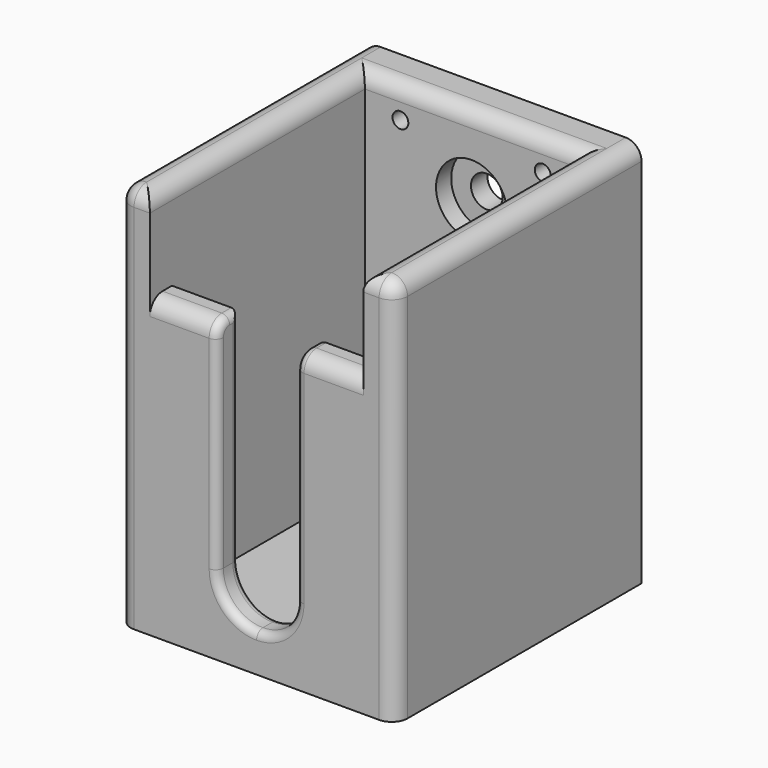
from build123d import *

# Parameters (mm, degrees)
F0_W           = 9
F0_H           = 7.5
F0_W_2         = 13.5
F0_H_2         = 34.5
F1_DEPTH       = 39
F2_DEPTH       = 34
F3_D           = 2
F3_DEPTH       = 40
F3_START       = 34
F3_TIP         = 0.600860619
F4_DEPTH       = 3.5
F5_R           = 1.99999
F7_D           = 4
F7_DEPTH       = 10
F7_CBORE_D     = 9
F7_CBORE_DEPTH = 2.4
F7_TIP         = 1.2017212381
F8_DEPTH       = 50
F9_R           = 1


# Not quite as in the source:
# - a fillet or chamfer is up to 0.001 mm smaller than in the source, because OpenCascade refuses the exact size


with BuildPart() as f1:
    # F0 (on Front) → F1 (new body)
    with BuildSketch(Plane.XZ):
        Polygon((13.5, 0), (0, 0), (-13.5, 0), (-13.5, 34.5), (-13.5, 36), (-13.5, 46), (-17.5, 46), (-17.5, 0), (-17.5, -3), (-13.5, -3), (13.5, -3), align=None)
        Polygon((13.5, 34.5), (13.5, 0), (13.5, -3), (17.5, -3), (17.5, 0), (17.5, 46), (13.5, 46), align=None)
        Polygon((-13.5, 0), (0, 0), (0, 34.5), (-9, 34.5), (-13.5, 34.5), align=None)
        Polygon((0, 42), (0, 34.5), (13.5, 34.5), (13.5, 46), (-13.5, 46), (-13.5, 36), (-13.5, 34.5), (-9, 34.5), (-9, 42), align=None)
        with Locations((-4.5, 38.25)):
            Rectangle(F0_W, F0_H)
        with Locations((6.75, 17.25)):
            Rectangle(F0_W_2, F0_H_2)
    extrude(amount=-F1_DEPTH)

    # F0 (on Front) → F2 (cut)
    with BuildSketch(Plane.XZ):
        Polygon((-13.5, 0), (0, 0), (0, 34.5), (-9, 34.5), (-13.5, 34.5), align=None)
        with Locations((6.75, 17.25)):
            Rectangle(F0_W_2, F0_H_2)
        Polygon((0, 42), (0, 34.5), (13.5, 34.5), (13.5, 46), (-13.5, 46), (-13.5, 36), (-13.5, 34.5), (-9, 34.5), (-9, 42), align=None)
        with Locations((-4.5, 38.25)):
            Rectangle(F0_W, F0_H)
    extrude(amount=-F2_DEPTH, mode=Mode.SUBTRACT)

    # F3
    # its depths count from where the whole tool has entered the part; down to there all is cleared
    with Locations(Plane.XZ.offset(-F3_START)):
        with Locations((-9, 42), (9, 42)):
            Hole(F3_D / 2, depth=F3_DEPTH)
            with Locations((0, 0, -(F3_DEPTH + F3_TIP / 2))):  # 118° drill point
                Cone(0, F3_D / 2, F3_TIP, mode=Mode.SUBTRACT)

    # F0 (on Front) → F4 (join)
    with BuildSketch(Plane.XZ):
        Polygon((-13.5, 0), (0, 0), (0, 34.5), (-9, 34.5), (-13.5, 34.5), align=None)
        with Locations((6.75, 17.25)):
            Rectangle(F0_W_2, F0_H_2)
    extrude(amount=-F4_DEPTH)

    # F5 (radius 2 in the source; OpenCascade refuses exactly that, so slightly less here)
    f5_edges = [f1.edges().sort_by_distance(p)[0] for p in [
        (-15.5, 0, 46),
        (-17.5, 0, 21.5),
        (17.5, 0, 21.5),
        (15.5, 0, 46),
        (-17.5, 19.5, 46),
        (17.5, 19.5, 46),
        (0, 34, 46),
        (13.5, 17, 46),
        (-13.5, 17, 46),
        (0, 0, 34.5),
    ]]
    fillet(f5_edges, radius=F5_R)

    # F7
    with Locations(Plane.XZ.offset(-34)):
        with Locations((0, 36), (0, 16)):
            CounterBoreHole(F7_D / 2, F7_CBORE_D / 2, F7_CBORE_DEPTH, depth=F7_DEPTH)
            with Locations((0, 0, -(F7_DEPTH + F7_TIP / 2))):  # 118° drill point
                Cone(0, F7_D / 2, F7_TIP, mode=Mode.SUBTRACT)

    # F6 (on face) → F8 (cut)
    with BuildSketch(Plane.XZ.offset(-34)):
        with BuildLine():
            ThreePointArc((-5, 6.8252934143), (-3.5355339059, 3.2897595084), (0, 1.8252934143))
            Line((0, 1.8252934143), (0, 6.8252934143))
            Line((0, 6.8252934143), (-5, 6.8252934143))
        make_face()
        with BuildLine():
            Line((0, 6.8252934143), (0, 1.8252934143))
            ThreePointArc((0, 1.8252934143), (3.5355339059, 3.2897595084), (5, 6.8252934143))
            ThreePointArc((5, 6.8252934143), (3.5355339059, 10.3608273202), (0, 11.8252934143))
            Line((0, 11.8252934143), (0, 6.8252934143))
        make_face()
        with BuildLine():
            Line((-5, 6.8252934143), (0, 6.8252934143))
            Line((0, 6.8252934143), (0, 11.8252934143))
            ThreePointArc((0, 11.8252934143), (-3.5355339059, 10.3608273202), (-5, 6.8252934143))
        make_face()
        with BuildLine():
            Line((-5, 35.0794121623), (-5, 6.8252934143))
            ThreePointArc((-5, 6.8252934143), (-3.5355339059, 10.3608273202), (0, 11.8252934143))
            Line((0, 11.8252934143), (0, 16))
            Line((0, 16), (0, 35.0794121623))
            Line((0, 35.0794121623), (-5, 35.0794121623))
        make_face()
        with BuildLine():
            ThreePointArc((0, 11.8252934143), (3.5355339059, 10.3608273202), (5, 6.8252934143))
            Line((5, 6.8252934143), (5, 35.0794121623))
            Line((5, 35.0794121623), (0, 35.0794121623))
            Line((0, 35.0794121623), (0, 16))
            Line((0, 16), (0, 11.8252934143))
        make_face()
    extrude(amount=F8_DEPTH, mode=Mode.SUBTRACT)

    # F9
    f9_edges = [f1.edges().sort_by_distance(p)[0] for p in [
        (5, 3.5, 20.662647),
        (5, 0, 19.662652),
        (0, 3.5, 1.825293),
    ]]
    fillet(f9_edges, radius=F9_R)


solid = f1.part
